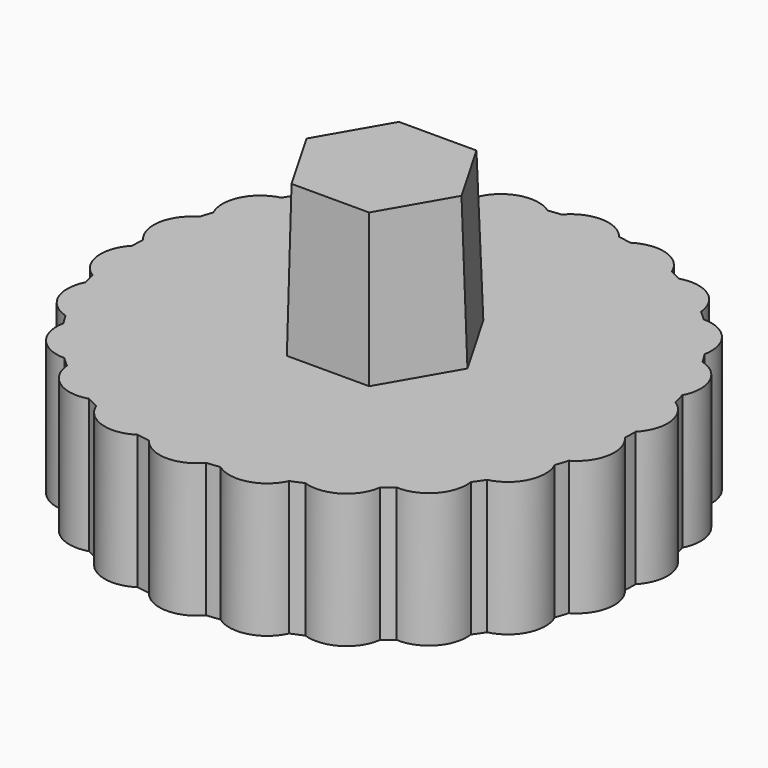
from build123d import *

# Parameters (mm, degrees)
F3_DEPTH = 8
F4_DEPTH = 8
F5_COUNT = 22


with BuildPart() as f3:
    # F2 (on offset) → F3 (new body)
    with BuildSketch(Plane.XY.offset(-9)):
        with BuildLine():
            ThreePointArc((14.5934619862, 3.4685540585), (-14.8980188245, -1.7461486487), (15, 0))
            ThreePointArc((15, 0), (14.8980188245, 1.7461486487), (14.5934619862, 3.4685540585))
        make_face()
        Polygon((-2.4537386441, -4.1687808289), (-4.9074772881, 0.0812191711), (-2.4537386441, 4.3312191711), (2.4537386441, 4.3312191711), (4.9074772881, 0.0812191711), (2.4537386441, -4.1687808289), align=None, mode=Mode.SUBTRACT)
        Polygon((-2.4537386441, 4.3312191711), (-4.9074772881, 0.0812191711), (-2.4537386441, -4.1687808289), (2.4537386441, -4.1687808289), (4.9074772881, 0.0812191711), (2.4537386441, 4.3312191711), align=None)
    extrude(amount=-F3_DEPTH)

    # F2 (on offset) → F4 (join, through all)
    with BuildSketch(Plane.XY.offset(-9)):
        with BuildLine():
            ThreePointArc((14.5934619862, 3.4685540585), (14.8980188245, 1.7461486487), (15, 0))
            ThreePointArc((15, 0), (15.6209528999, 1.8308814158), (14.5934619862, 3.4685540585))
        make_face()
    extrude(amount=-F4_DEPTH)

    # F5: F3 ×22 about axis
    f5_axis = Axis((0, 0, -9), (0, 0, 1))


with BuildPart() as f3_1:
    add(f3.part)
    for i in range(1, F5_COUNT):
        add(f3.part.rotate(f5_axis, i * 360 / F5_COUNT))

    # F0 (on Top) → F6 section 0
    with BuildSketch(Plane.XY):
        Polygon((-4.6188021535, 0), (-2.3094010768, -4), (2.3094010768, -4), (4.6188021535, 0), (2.3094010768, 4), (-2.3094010768, 4), align=None)
    # F2 (on offset) → F6 section 1
    with BuildSketch(Plane.XY.offset(-9)):
        Polygon((-2.4537386441, 4.3312191711), (-4.9074772881, 0.0812191711), (-2.4537386441, -4.1687808289), (2.4537386441, -4.1687808289), (4.9074772881, 0.0812191711), (2.4537386441, 4.3312191711), align=None)
    loft()


solid = f3_1.part
